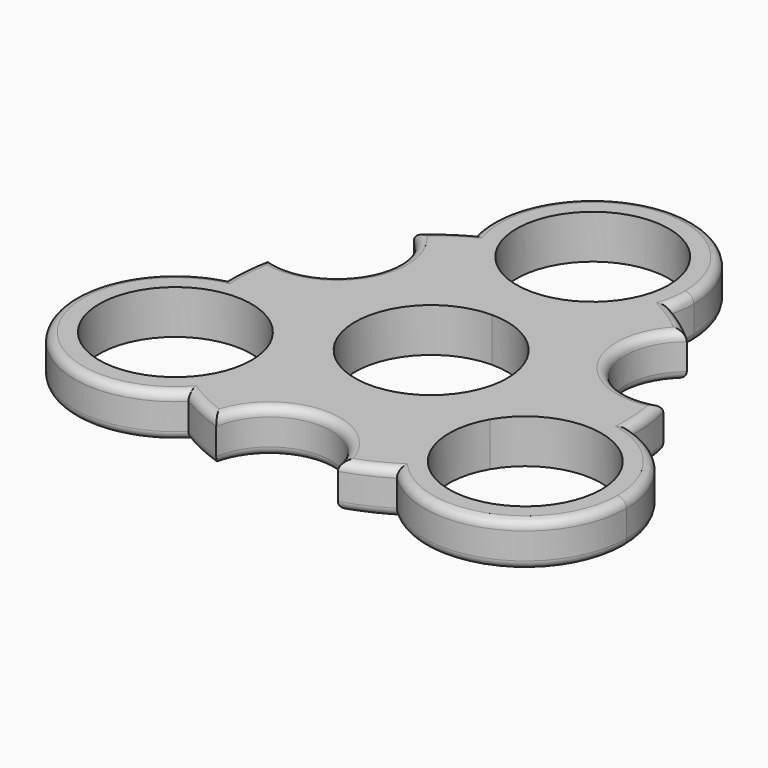
from build123d import *

# Parameters (mm, degrees)
F1_DEPTH = 6.35
F2_R     = 1.27


# Not quite as in the source:
# - ends of sketch curves that miss each other by under 0.0002 mm in the source are joined


with BuildPart() as f1:
    # F0 (on Top) → F1 (new body)
    with BuildSketch(Plane.XY):
        with BuildLine():
            ThreePointArc((-14.1412304428, 25.55875), (-8.9436994156, 17.6637336874), (1.95e-08, 14.605))
            ThreePointArc((1.95e-08, 14.605), (8.943699431, 17.6637336993), (14.1412304428, 25.55875))
            ThreePointArc((14.1412304428, 25.55875), (14.488593714, 27.3697073083), (14.605, 29.21))
            ThreePointArc((14.605, 29.21), (-1.8402926917, 43.698593714), (-14.1412304428, 25.55875))
        make_face()
        with BuildLine():
            ThreePointArc((11.0109, 29.21), (7.785882057, 21.424117943), (0, 18.1991))
            ThreePointArc((0, 18.1991), (-7.785882057, 36.995882057), (11.0109, 29.21))
        make_face(mode=Mode.SUBTRACT)
        with BuildLine():
            ThreePointArc((-10.6916020445, -14.605), (-11.1892553654, -10.8249477946), (-12.6483010757, -7.3024999074))
            ThreePointArc((-12.6483010757, -7.3024999074), (-19.7690918652, -1.086395922), (-29.2051420104, -0.5327101957))
            ThreePointArc((-29.2051420104, -0.5327101957), (-37.9449030668, -21.9075), (-15.0639115676, -25.0260398043))
            ThreePointArc((-15.0639115676, -25.0260398043), (-11.8289654773, -20.2555566356), (-10.6916020445, -14.605))
        make_face()
        with BuildLine():
            ThreePointArc((-14.2857020445, -14.605), (-35.9323147252, -17.4548306237), (-15.760882926, -9.09955))
            ThreePointArc((-15.760882926, -9.09955), (-14.6608893639, -11.7551693763), (-14.2857020445, -14.605))
        make_face(mode=Mode.SUBTRACT)
        with BuildLine():
            ThreePointArc((29.2051420104, -0.5327101957), (19.7690918491, -1.0863959286), (12.6483010583, -7.3024999376))
            ThreePointArc((12.6483010583, -7.3024999376), (10.8253923876, -16.5773377154), (15.0639115676, -25.0260398043))
            ThreePointArc((15.0639115676, -25.0260398043), (30.9471586801, -28.0726365673), (39.9016020445, -14.605))
            ThreePointArc((39.9016020445, -14.605), (36.9239459201, -5.7669629216), (29.2051420104, -0.5327101957))
        make_face()
        with BuildLine():
            ThreePointArc((36.3075020445, -14.605), (22.4467714208, -25.2407126807), (15.760882926, -9.09955))
            ThreePointArc((15.760882926, -9.09955), (28.1464326683, -3.9692873193), (36.3075020445, -14.605))
        make_face(mode=Mode.SUBTRACT)
        with BuildLine():
            ThreePointArc((-12.6483010757, -7.3024999074), (-12.6483009907, 7.3025000547), (1.95e-08, 14.605))
            ThreePointArc((1.95e-08, 14.605), (-8.9436994156, 17.6637336874), (-14.1412304428, 25.55875))
            ThreePointArc((-14.1412304428, 25.55875), (-17.0554148392, 23.7136442721), (-19.7317879462, 21.5378885791))
            ThreePointArc((-19.7317879462, 21.5378885791), (-17.5976362049, 10.16), (-28.5182526265, 6.3192853339))
            ThreePointArc((-28.5182526265, 6.3192853339), (-29.0643257755, 2.9136003868), (-29.2051420104, -0.5327101957))
            ThreePointArc((-29.2051420104, -0.5327101957), (-19.7690918652, -1.086395922), (-12.6483010757, -7.3024999074))
        make_face()
        with BuildLine():
            ThreePointArc((15.0639115676, -25.0260398043), (10.8253923876, -16.5773377154), (12.6483010583, -7.3024999376))
            ThreePointArc((12.6483010583, -7.3024999376), (-1.74e-08, -14.605), (-12.6483010757, -7.3024999074))
            ThreePointArc((-12.6483010757, -7.3024999074), (-11.1892553654, -10.8249477946), (-10.6916020445, -14.605))
            ThreePointArc((-10.6916020445, -14.605), (-11.8289654773, -20.2555566356), (-15.0639115676, -25.0260398043))
            ThreePointArc((-15.0639115676, -25.0260398043), (-12.0089109363, -26.6272446589), (-8.7864646803, -27.857173913))
            ThreePointArc((-8.7864646803, -27.857173913), (0, -20.32), (8.7864646803, -27.857173913))
            ThreePointArc((8.7864646803, -27.857173913), (12.0089109363, -26.6272446589), (15.0639115676, -25.0260398043))
        make_face()
        with BuildLine():
            ThreePointArc((14.1412304428, 25.55875), (8.943699431, 17.6637336993), (1.95e-08, 14.605))
            ThreePointArc((1.95e-08, 14.605), (10.3272945461, 10.3272945323), (14.605, 0))
            ThreePointArc((14.605, 0), (14.1073467023, -3.7800521189), (12.6483010583, -7.3024999376))
            ThreePointArc((12.6483010583, -7.3024999376), (19.7690918491, -1.0863959286), (29.2051420104, -0.5327101957))
            ThreePointArc((29.2051420104, -0.5327101957), (29.0643257755, 2.9136003868), (28.5182526265, 6.3192853339))
            ThreePointArc((28.5182526265, 6.3192853339), (17.5976362049, 10.16), (19.7317879462, 21.5378885791))
            ThreePointArc((19.7317879462, 21.5378885791), (17.0554148392, 23.7136442721), (14.1412304428, 25.55875))
        make_face()
        with BuildLine():
            ThreePointArc((-9.5357191185, -5.50545), (-9.5357191185, 5.50545), (0, 11.0109))
            Line((0, 11.0109), (0, 14.605))
            ThreePointArc((0, 14.605), (-12.6483009907, 7.3025000547), (-12.6483010757, -7.3024999074))
            Line((-12.6483010757, -7.3024999074), (-9.5357191185, -5.50545))
        make_face()
        with BuildLine():
            Line((12.6483010223, -7.3025), (9.5357191185, -5.50545))
            ThreePointArc((9.5357191185, -5.50545), (0, -11.0109), (-9.5357191185, -5.50545))
            Line((-9.5357191185, -5.50545), (-12.6483010223, -7.3025))
            ThreePointArc((-12.6483010223, -7.3025), (-1.74e-08, -14.605), (12.6483010223, -7.3025))
        make_face()
        with BuildLine():
            ThreePointArc((0, 11.0109), (7.785882057, 7.785882057), (11.0109, 0))
            ThreePointArc((11.0109, 0), (10.6357126807, -2.8498306237), (9.5357191185, -5.50545))
            Line((9.5357191185, -5.50545), (12.6483010223, -7.3025))
            ThreePointArc((12.6483010583, -7.3024999376), (14.1073467023, -3.7800521189), (14.605, 0))
            ThreePointArc((14.605, 0), (10.3272945461, 10.3272945323), (1.95e-08, 14.605))
            Line((0, 14.605), (0, 11.0109))
        make_face()
    extrude(amount=F1_DEPTH)

    # F2
    f2_edges = [f1.edges().sort_by_distance(p)[0] for p in [
        (0, 43.815, 6.35),
        (-17.597636, 10.16, 6.35),
        (-37.944903, -21.9075, 6.35),
        (-29.064326, 2.9136, 6.35),
        (-12.008911, -26.627245, 6.35),
        (0, -20.32, 6.35),
        (12.008911, -26.627245, 6.35),
        (37.944903, -21.9075, 6.35),
        (29.064326, 2.9136, 6.35),
        (17.597636, 10.16, 6.35),
        (17.055415, 23.713644, 6.35),
        (-17.055415, 23.713644, 6.35),
        (0, 43.815, 0),
        (17.055415, 23.713644, 0),
        (17.597636, 10.16, 0),
        (29.064326, 2.9136, 0),
        (37.944903, -21.9075, 0),
        (12.008911, -26.627245, 0),
        (0, -20.32, 0),
        (-12.008911, -26.627245, 0),
        (-37.944903, -21.9075, 0),
        (-29.064326, 2.9136, 0),
        (-17.055415, 23.713644, 0),
        (-17.597636, 10.16, 0),
    ]]
    fillet(f2_edges, radius=F2_R)


solid = f1.part
